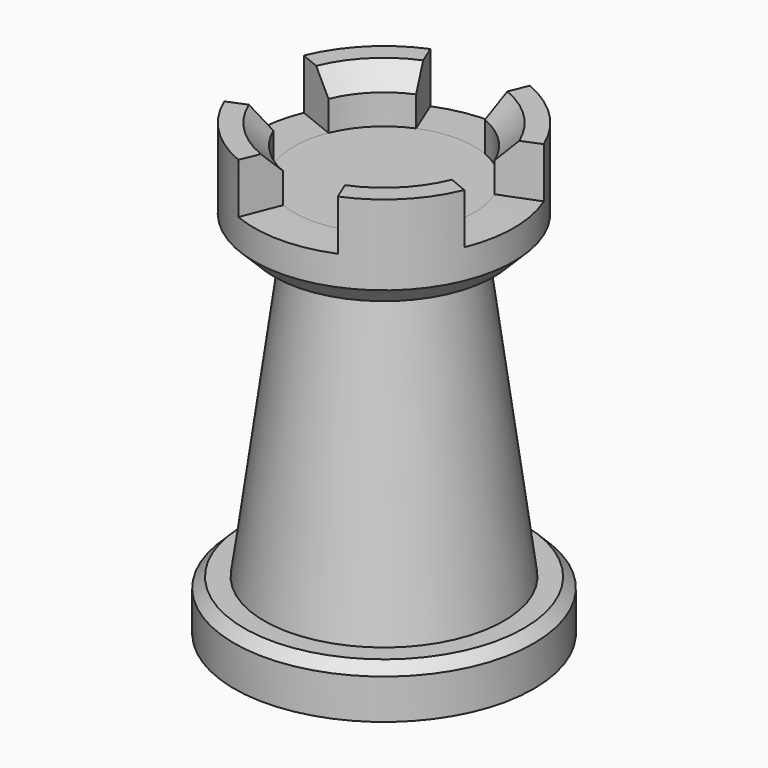
from build123d import *

# Parameters (mm, degrees)
F0_R            = 9.525
F1_DEPTH        = 3.175
F2_SIZE         = 0.635
F6_ANGLE_BACK   = 22.5
F6_ANGLE        = 45
F6_COPIES_COUNT = 4
F7_SIZE         = 1.27
F8_SIZE         = 1.27


# Not quite as in the source:
# - a pattern or mirror of a feature is missing from the dataset's text; its kind, count and spacing are read off the source's solid


with BuildPart() as f1:
    # F0 (on Top) → F1 (new body)
    with BuildSketch(Plane.XY):
        Circle(F0_R)
    extrude(amount=F1_DEPTH)

    # F2
    f2_edges = [f1.edges().sort_by_distance(p)[0] for p in [
        (-9.525, 0, 3.175),
    ]]
    chamfer(f2_edges, length=F2_SIZE)

    # F3 (on Front) → F4 (revolve)
    with BuildSketch(Plane.XZ):
        Polygon((-5.08, 22.225), (-7.62, 3.175), (0, 3.175), (0, 22.225), (0, 25.4), (-5.715, 25.4), (-5.715, 28.575), (-8.255, 28.575), (-8.255, 22.225), align=None)
    revolve(axis=Axis((0, 0, 12.7), (0, 0, 1)))

    # F5 (on Right) → F6 (revolve, cut)
    with BuildSketch(Plane.YZ, mode=Mode.PRIVATE) as f6_sk:
        Polygon((-5.715, 25.4), (-5.715, 28.575), (-8.255, 28.575), (-8.255, 25.3708213568), align=None)
    f6 = revolve(f6_sk.sketch.rotate(Axis((0, 0, 12.7), (0, 0, -1)), -F6_ANGLE_BACK), axis=Axis((0, 0, 12.7), (0, 0, -1)), revolution_arc=F6_ANGLE, mode=Mode.SUBTRACT)

    # F6_copies: F6 ×4 about axis
    f6_copies_axis = Axis((0, 0, 0), (0, 0, 1))
    for i in range(1, F6_COPIES_COUNT):
        add(f6.rotate(f6_copies_axis, i * 360 / F6_COPIES_COUNT), mode=Mode.SUBTRACT)

    # F7
    f7_edges = [f1.edges().sort_by_distance(p)[0] for p in [
        (8.255, 0, 22.225),
    ]]
    chamfer(f7_edges, length=F7_SIZE)

    # F8
    f8_edges = [f1.edges().sort_by_distance(p)[0] for p in [
        (-4.041115, -4.041115, 28.575),
        (-4.041115, 4.041115, 28.575),
        (4.041115, -4.041115, 28.575),
        (4.041115, 4.041115, 28.575),
    ]]
    chamfer(f8_edges, length=F8_SIZE)


solid = f1.part
